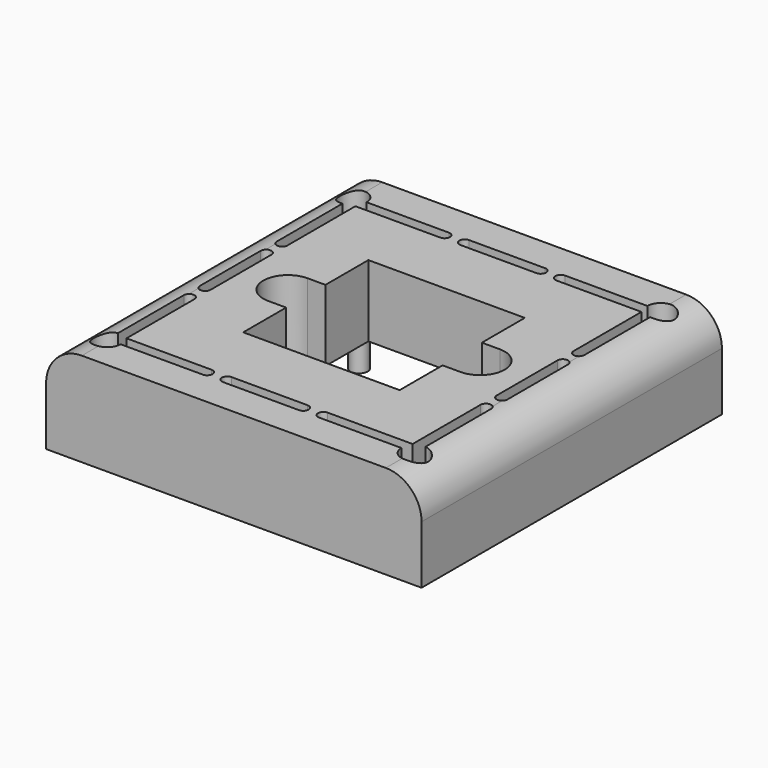
from build123d import *

# Parameters (mm, degrees)
F0_W        = 39
F0_H        = 39
F0_R        = 0.975
F1_DEPTH    = 9
F2_T1_DEPTH = 62
F3_DEPTH    = 5.5
F4_DEPTH    = 1.5
F5_DEPTH    = 2.5
F6_DEPTH    = 1.5
F7_DEPTH    = 5
F8_DEPTH    = 1


# Not quite as in the source:
# - a fillet or chamfer that OpenCascade refuses, or shapes differently, is made with other operations: its cross-section is extruded or revolved along the edge and cut away or added


with BuildPart() as f1:
    # F0 (on Top) → F1 (new body)
    with BuildSketch(Plane.XY):
        Polygon((-2.625, 21), (-21, 21), (-21, -21), (-2.625, -21), (2.625, -21), (21, -21), (21, 21), (2.625, 21), align=None)
        Rectangle(F0_W, F0_H, mode=Mode.SUBTRACT)
        Rectangle(F0_W, F0_H)
        with BuildLine():
            ThreePointArc((16, 4.25), (16.6, 4.85), (17.2, 4.25))
            Line((17.2, 4.25), (17.2, -4.25))
            ThreePointArc((17.2, -4.25), (16.6, -4.85), (16, -4.25))
            Line((16, -4.25), (16, -6.5))
            ThreePointArc((16, -6.5), (16.6, -5.9), (17.2, -6.5))
            Line((17.2, -6.5), (17.2, -15.7))
            ThreePointArc((17.2, -15.7), (18.2606601718, -18.2606601718), (15.7, -17.2))
            Line((15.7, -17.2), (6.5, -17.2))
            ThreePointArc((6.5, -17.2), (5.9, -16.6), (6.5, -16))
            Line((6.5, -16), (4.25, -16))
            ThreePointArc((4.25, -16), (4.85, -16.6), (4.25, -17.2))
            Line((4.25, -17.2), (-4.25, -17.2))
            ThreePointArc((-4.25, -17.2), (-4.85, -16.6), (-4.25, -16))
            Line((-4.25, -16), (-6.5, -16))
            ThreePointArc((-6.5, -16), (-5.9, -16.6), (-6.5, -17.2))
            Line((-6.5, -17.2), (-15.7, -17.2))
            ThreePointArc((-15.7, -17.2), (-18.2606601718, -18.2606601718), (-17.2, -15.7))
            Line((-17.2, -15.7), (-17.2, -6.5))
            ThreePointArc((-17.2, -6.5), (-16.6, -5.9), (-16, -6.5))
            Line((-16, -6.5), (-16, -4.25))
            ThreePointArc((-16, -4.25), (-16.6, -4.85), (-17.2, -4.25))
            Line((-17.2, -4.25), (-17.2, 4.25))
            ThreePointArc((-17.2, 4.25), (-16.6, 4.85), (-16, 4.25))
            Line((-16, 4.25), (-16, 6.5))
            ThreePointArc((-16, 6.5), (-16.6, 5.9), (-17.2, 6.5))
            Line((-17.2, 6.5), (-17.2, 15.7))
            ThreePointArc((-17.2, 15.7), (-18.2606601718, 18.2606601718), (-15.7, 17.2))
            Line((-15.7, 17.2), (-6.5, 17.2))
            ThreePointArc((-6.5, 17.2), (-5.9, 16.6), (-6.5, 16))
            Line((-6.5, 16), (-4.25, 16))
            ThreePointArc((-4.25, 16), (-4.85, 16.6), (-4.25, 17.2))
            Line((-4.25, 17.2), (4.25, 17.2))
            ThreePointArc((4.25, 17.2), (4.85, 16.6), (4.25, 16))
            Line((4.25, 16), (6.5, 16))
            ThreePointArc((6.5, 16), (5.9, 16.6), (6.5, 17.2))
            Line((6.5, 17.2), (15.7, 17.2))
            ThreePointArc((15.7, 17.2), (18.2606601718, 18.2606601718), (17.2, 15.7))
            Line((17.2, 15.7), (17.2, 6.5))
            ThreePointArc((17.2, 6.5), (16.6, 5.9), (16, 6.5))
            Line((16, 6.5), (16, 4.25))
        make_face(mode=Mode.SUBTRACT)
        Polygon((16, -4.25), (16, 4.25), (16, 6.5), (16, 16), (6.5, 16), (4.25, 16), (-4.25, 16), (-6.5, 16), (-16, 16), (-16, 6.5), (-16, 4.25), (-16, -4.25), (-16, -6.5), (-16, -16), (-6.5, -16), (-4.25, -16), (4.25, -16), (6.5, -16), (16, -16), (16, -6.5), align=None)
        with Locations((-14, -14)):
            Circle(F0_R, mode=Mode.SUBTRACT)
        with Locations((14, -14)):
            Circle(F0_R, mode=Mode.SUBTRACT)
        with Locations((-14, 14)):
            Circle(F0_R, mode=Mode.SUBTRACT)
        Polygon((-8.75, 14), (0, 14), (0, 10.75), (-8.75, 10.75), (-9.75, 10.75), (-9.75, 14), align=None, mode=Mode.SUBTRACT)
        with BuildLine():
            Line((-8.75, 8.75), (8.75, 8.75))
            Line((8.75, 8.75), (8.75, 2.75))
            Line((8.75, 2.75), (10.75, 2.75))
            ThreePointArc((10.75, 2.75), (13.5, 0), (10.75, -2.75))
            Line((10.75, -2.75), (8.75, -2.75))
            Line((8.75, -2.75), (8.75, -8.75))
            Line((8.75, -8.75), (-8.75, -8.75))
            Line((-8.75, -8.75), (-8.75, -2.75))
            Line((-8.75, -2.75), (-10.75, -2.75))
            ThreePointArc((-10.75, -2.75), (-13.5, 0), (-10.75, 2.75))
            Line((-10.75, 2.75), (-8.75, 2.75))
            Line((-8.75, 2.75), (-8.75, 8.75))
        make_face(mode=Mode.SUBTRACT)
        Polygon((10.75, 3.8126846775), (10.75, 8.75), (10.75, 9.75), (14, 9.75), (14, 8.75), (14, 3.8126846775), align=None, mode=Mode.SUBTRACT)
        with Locations((14, 14)):
            Circle(F0_R, mode=Mode.SUBTRACT)
        Polygon((0, 10.75), (0, 14), (-8.75, 14), (-9.75, 14), (-9.75, 10.75), (-8.75, 10.75), align=None)
        Polygon((10.75, 9.75), (10.75, 8.75), (10.75, 3.8126846775), (14, 3.8126846775), (14, 8.75), (14, 9.75), align=None)
        with Locations((14, -14)):
            Circle(F0_R)
        with Locations((-14, -14)):
            Circle(F0_R)
        with Locations((-14, 14)):
            Circle(F0_R)
        with Locations((14, 14)):
            Circle(F0_R)
    extrude(amount=F1_DEPTH)

    # F2: fillet of radius 4 on 2 edges, made by hand

    # F2_s2 → F2_t1 (cut)
    with BuildSketch(Plane.XZ.offset(-31)):
        with BuildLine():
            ThreePointArc((-21, 5), (-19.8284271247, 7.8284271247), (-17, 9))
            Line((-17, 9), (-21, 9))
            Line((-21, 9), (-21, 5))
        make_face()
        with BuildLine():
            ThreePointArc((21, 5), (19.8284271247, 7.8284271247), (17, 9))
            Line((17, 9), (21, 9))
            Line((21, 9), (21, 5))
        make_face()
    extrude(amount=F2_T1_DEPTH, mode=Mode.SUBTRACT)

    # F0 (on Top) → F3 (join)
    with BuildSketch(Plane.XY):
        with Locations((-14, -14)):
            Circle(F0_R)
        with Locations((14, -14)):
            Circle(F0_R)
        with Locations((-14, 14)):
            Circle(F0_R)
        with Locations((14, 14)):
            Circle(F0_R)
    extrude(amount=-F3_DEPTH)

    # F0 (on Top) → F4 (join)
    with BuildSketch(Plane.XY):
        Rectangle(F0_W, F0_H)
        with BuildLine():
            ThreePointArc((16, 4.25), (16.6, 4.85), (17.2, 4.25))
            Line((17.2, 4.25), (17.2, -4.25))
            ThreePointArc((17.2, -4.25), (16.6, -4.85), (16, -4.25))
            Line((16, -4.25), (16, -6.5))
            ThreePointArc((16, -6.5), (16.6, -5.9), (17.2, -6.5))
            Line((17.2, -6.5), (17.2, -15.7))
            ThreePointArc((17.2, -15.7), (18.2606601718, -18.2606601718), (15.7, -17.2))
            Line((15.7, -17.2), (6.5, -17.2))
            ThreePointArc((6.5, -17.2), (5.9, -16.6), (6.5, -16))
            Line((6.5, -16), (4.25, -16))
            ThreePointArc((4.25, -16), (4.85, -16.6), (4.25, -17.2))
            Line((4.25, -17.2), (-4.25, -17.2))
            ThreePointArc((-4.25, -17.2), (-4.85, -16.6), (-4.25, -16))
            Line((-4.25, -16), (-6.5, -16))
            ThreePointArc((-6.5, -16), (-5.9, -16.6), (-6.5, -17.2))
            Line((-6.5, -17.2), (-15.7, -17.2))
            ThreePointArc((-15.7, -17.2), (-18.2606601718, -18.2606601718), (-17.2, -15.7))
            Line((-17.2, -15.7), (-17.2, -6.5))
            ThreePointArc((-17.2, -6.5), (-16.6, -5.9), (-16, -6.5))
            Line((-16, -6.5), (-16, -4.25))
            ThreePointArc((-16, -4.25), (-16.6, -4.85), (-17.2, -4.25))
            Line((-17.2, -4.25), (-17.2, 4.25))
            ThreePointArc((-17.2, 4.25), (-16.6, 4.85), (-16, 4.25))
            Line((-16, 4.25), (-16, 6.5))
            ThreePointArc((-16, 6.5), (-16.6, 5.9), (-17.2, 6.5))
            Line((-17.2, 6.5), (-17.2, 15.7))
            ThreePointArc((-17.2, 15.7), (-18.2606601718, 18.2606601718), (-15.7, 17.2))
            Line((-15.7, 17.2), (-6.5, 17.2))
            ThreePointArc((-6.5, 17.2), (-5.9, 16.6), (-6.5, 16))
            Line((-6.5, 16), (-4.25, 16))
            ThreePointArc((-4.25, 16), (-4.85, 16.6), (-4.25, 17.2))
            Line((-4.25, 17.2), (4.25, 17.2))
            ThreePointArc((4.25, 17.2), (4.85, 16.6), (4.25, 16))
            Line((4.25, 16), (6.5, 16))
            ThreePointArc((6.5, 16), (5.9, 16.6), (6.5, 17.2))
            Line((6.5, 17.2), (15.7, 17.2))
            ThreePointArc((15.7, 17.2), (18.2606601718, 18.2606601718), (17.2, 15.7))
            Line((17.2, 15.7), (17.2, 6.5))
            ThreePointArc((17.2, 6.5), (16.6, 5.9), (16, 6.5))
            Line((16, 6.5), (16, 4.25))
        make_face(mode=Mode.SUBTRACT)
    extrude(amount=-F4_DEPTH)

    # F5 (cut): a face of the model
    f5_faces = [f1.faces().sort_by_distance(p)[0] for p in [
        (-18.9484567107, 0, -1.5),
    ]]
    extrude(f5_faces, amount=-F5_DEPTH, mode=Mode.SUBTRACT)

    # F0 (on Top) → F6 (join)
    with BuildSketch(Plane.XY):
        Polygon((-2.625, 21), (-21, 21), (-21, -21), (-2.625, -21), (2.625, -21), (21, -21), (21, 21), (2.625, 21), align=None)
        Rectangle(F0_W, F0_H, mode=Mode.SUBTRACT)
    extrude(amount=-F6_DEPTH)

    # F0 (on Top) → F7 (cut)
    with BuildSketch(Plane.XY):
        Polygon((10.75, 9.75), (10.75, 8.75), (10.75, 3.8126846775), (14, 3.8126846775), (14, 8.75), (14, 9.75), align=None)
        Polygon((0, 10.75), (0, 14), (-8.75, 14), (-9.75, 14), (-9.75, 10.75), (-8.75, 10.75), align=None)
    extrude(amount=F7_DEPTH, mode=Mode.SUBTRACT)

    # F0 (on Top) → F8 (cut)
    with BuildSketch(Plane.XY):
        Polygon((16, -4.25), (16, 4.25), (16, 6.5), (16, 16), (6.5, 16), (4.25, 16), (-4.25, 16), (-6.5, 16), (-16, 16), (-16, 6.5), (-16, 4.25), (-16, -4.25), (-16, -6.5), (-16, -16), (-6.5, -16), (-4.25, -16), (4.25, -16), (6.5, -16), (16, -16), (16, -6.5), align=None)
        with Locations((-14, -14)):
            Circle(F0_R, mode=Mode.SUBTRACT)
        with Locations((14, -14)):
            Circle(F0_R, mode=Mode.SUBTRACT)
        with Locations((-14, 14)):
            Circle(F0_R, mode=Mode.SUBTRACT)
        Polygon((-8.75, 14), (0, 14), (0, 10.75), (-8.75, 10.75), (-9.75, 10.75), (-9.75, 14), align=None, mode=Mode.SUBTRACT)
        with BuildLine():
            Line((-8.75, 8.75), (8.75, 8.75))
            Line((8.75, 8.75), (8.75, 2.75))
            Line((8.75, 2.75), (10.75, 2.75))
            ThreePointArc((10.75, 2.75), (13.5, 0), (10.75, -2.75))
            Line((10.75, -2.75), (8.75, -2.75))
            Line((8.75, -2.75), (8.75, -8.75))
            Line((8.75, -8.75), (-8.75, -8.75))
            Line((-8.75, -8.75), (-8.75, -2.75))
            Line((-8.75, -2.75), (-10.75, -2.75))
            ThreePointArc((-10.75, -2.75), (-13.5, 0), (-10.75, 2.75))
            Line((-10.75, 2.75), (-8.75, 2.75))
            Line((-8.75, 2.75), (-8.75, 8.75))
        make_face(mode=Mode.SUBTRACT)
        Polygon((10.75, 3.8126846775), (10.75, 8.75), (10.75, 9.75), (14, 9.75), (14, 8.75), (14, 3.8126846775), align=None, mode=Mode.SUBTRACT)
        with Locations((14, 14)):
            Circle(F0_R, mode=Mode.SUBTRACT)
    extrude(amount=F8_DEPTH, mode=Mode.SUBTRACT)


solid = f1.part
